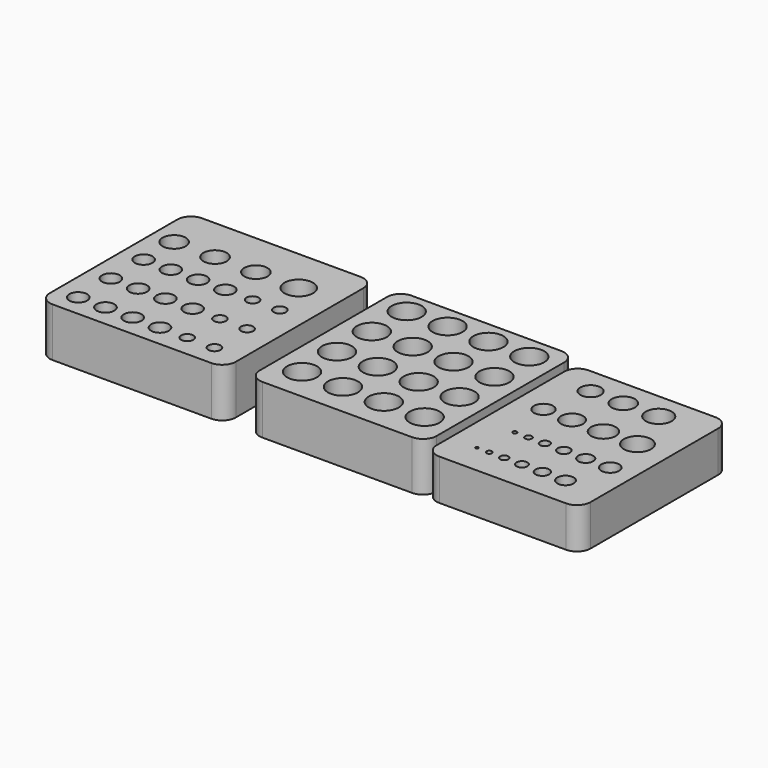
from build123d import *

# Parameters (mm, degrees)
F0_R     = 0.5
F0_R_2   = 1
F0_R_3   = 1.5
F0_R_4   = 2
F0_R_5   = 0.75
F0_R_6   = 1.25
F0_R_7   = 1.75
F0_R_8   = 2.5
F0_R_9   = 3
F0_R_10  = 2.25
F0_R_11  = 2.75
F0_R_12  = 3.25
F0_R_13  = 3.5
F0_R_14  = 4
F0_R_15  = 3.75
F0_R_16  = 4.25
F0_R_17  = 4.5
F0_R_18  = 5
F0_R_19  = 4.75
F1_DEPTH = 12
F2_DEPTH = 3
F3_R     = 5.5
F4_DEPTH = 15
F5_DEPTH = 3
F6_R     = 3.25
F6_R_2   = 2.25
F6_R_3   = 4.25
F6_R_4   = 5.25
F7_DEPTH = 15
F8_DEPTH = 3


with BuildPart() as f1:
    # F0 (on Top) → F1 (new body)
    with BuildSketch(Plane.XY):
        with BuildLine():
            Line((51.5, 68.5), (5, 68.5))
            ThreePointArc((5, 68.5), (1.4644660941, 67.0355339059), (0, 63.5))
            Line((0, 63.5), (0, 5))
            ThreePointArc((0, 5), (1.4644660941, 1.4644660941), (5, 0))
            Line((5, 0), (51.5, 0))
            ThreePointArc((51.5, 0), (55.0355339059, 1.4644660941), (56.5, 5))
            Line((56.5, 5), (56.5, 63.5))
            ThreePointArc((56.5, 63.5), (55.0355339059, 67.0355339059), (51.5, 68.5))
        make_face()
        with Locations((10, 11)):
            Circle(F0_R, mode=Mode.SUBTRACT)
        with Locations((14.5, 11)):
            Circle(F0_R_2, mode=Mode.SUBTRACT)
        with Locations((20, 11)):
            Circle(F0_R_3, mode=Mode.SUBTRACT)
        with Locations((26.5, 11)):
            Circle(F0_R_4, mode=Mode.SUBTRACT)
        with Locations((12.5, 25.25)):
            Circle(F0_R_5, mode=Mode.SUBTRACT)
        with Locations((17.5, 25.25)):
            Circle(F0_R_6, mode=Mode.SUBTRACT)
        with Locations((23.5, 25.25)):
            Circle(F0_R_7, mode=Mode.SUBTRACT)
        with Locations((34, 11)):
            Circle(F0_R_8, mode=Mode.SUBTRACT)
        with Locations((42.5, 11)):
            Circle(F0_R_9, mode=Mode.SUBTRACT)
        with Locations((30.5, 25.25)):
            Circle(F0_R_10, mode=Mode.SUBTRACT)
        with Locations((38.5, 25.25)):
            Circle(F0_R_11, mode=Mode.SUBTRACT)
        with Locations((47.5, 25.25)):
            Circle(F0_R_12, mode=Mode.SUBTRACT)
        with Locations((10, 41.5)):
            Circle(F0_R_13, mode=Mode.SUBTRACT)
        with Locations((20.5, 41.5)):
            Circle(F0_R_14, mode=Mode.SUBTRACT)
        with Locations((13.5, 58.75)):
            Circle(F0_R_15, mode=Mode.SUBTRACT)
        with Locations((25.5, 58.75)):
            Circle(F0_R_16, mode=Mode.SUBTRACT)
        with Locations((32, 41.5)):
            Circle(F0_R_17, mode=Mode.SUBTRACT)
        with Locations((44.5, 41.5)):
            Circle(F0_R_18, mode=Mode.SUBTRACT)
        with Locations((38.5, 58.75)):
            Circle(F0_R_19, mode=Mode.SUBTRACT)
    extrude(amount=F1_DEPTH)

    # F0 (on Top) → F2 (join)
    with BuildSketch(Plane.XY):
        with BuildLine():
            Line((51.5, 68.5), (5, 68.5))
            ThreePointArc((5, 68.5), (1.4644660941, 67.0355339059), (0, 63.5))
            Line((0, 63.5), (0, 5))
            ThreePointArc((0, 5), (1.4644660941, 1.4644660941), (5, 0))
            Line((5, 0), (51.5, 0))
            ThreePointArc((51.5, 0), (55.0355339059, 1.4644660941), (56.5, 5))
            Line((56.5, 5), (56.5, 63.5))
            ThreePointArc((56.5, 63.5), (55.0355339059, 67.0355339059), (51.5, 68.5))
        make_face()
        with Locations((10, 11)):
            Circle(F0_R, mode=Mode.SUBTRACT)
        with Locations((14.5, 11)):
            Circle(F0_R_2, mode=Mode.SUBTRACT)
        with Locations((20, 11)):
            Circle(F0_R_3, mode=Mode.SUBTRACT)
        with Locations((26.5, 11)):
            Circle(F0_R_4, mode=Mode.SUBTRACT)
        with Locations((12.5, 25.25)):
            Circle(F0_R_5, mode=Mode.SUBTRACT)
        with Locations((17.5, 25.25)):
            Circle(F0_R_6, mode=Mode.SUBTRACT)
        with Locations((23.5, 25.25)):
            Circle(F0_R_7, mode=Mode.SUBTRACT)
        with Locations((34, 11)):
            Circle(F0_R_8, mode=Mode.SUBTRACT)
        with Locations((42.5, 11)):
            Circle(F0_R_9, mode=Mode.SUBTRACT)
        with Locations((30.5, 25.25)):
            Circle(F0_R_10, mode=Mode.SUBTRACT)
        with Locations((38.5, 25.25)):
            Circle(F0_R_11, mode=Mode.SUBTRACT)
        with Locations((47.5, 25.25)):
            Circle(F0_R_12, mode=Mode.SUBTRACT)
        with Locations((10, 41.5)):
            Circle(F0_R_13, mode=Mode.SUBTRACT)
        with Locations((20.5, 41.5)):
            Circle(F0_R_14, mode=Mode.SUBTRACT)
        with Locations((13.5, 58.75)):
            Circle(F0_R_15, mode=Mode.SUBTRACT)
        with Locations((25.5, 58.75)):
            Circle(F0_R_16, mode=Mode.SUBTRACT)
        with Locations((32, 41.5)):
            Circle(F0_R_17, mode=Mode.SUBTRACT)
        with Locations((44.5, 41.5)):
            Circle(F0_R_18, mode=Mode.SUBTRACT)
        with Locations((38.5, 58.75)):
            Circle(F0_R_19, mode=Mode.SUBTRACT)
        with Locations((44.5, 41.5)):
            Circle(F0_R_18)
        with Locations((38.5, 58.75)):
            Circle(F0_R_19)
        with Locations((32, 41.5)):
            Circle(F0_R_17)
        with Locations((25.5, 58.75)):
            Circle(F0_R_16)
        with Locations((20.5, 41.5)):
            Circle(F0_R_14)
        with Locations((13.5, 58.75)):
            Circle(F0_R_15)
        with Locations((10, 41.5)):
            Circle(F0_R_13)
        with Locations((47.5, 25.25)):
            Circle(F0_R_12)
        with Locations((42.5, 11)):
            Circle(F0_R_9)
        with Locations((38.5, 25.25)):
            Circle(F0_R_11)
        with Locations((34, 11)):
            Circle(F0_R_8)
        with Locations((30.5, 25.25)):
            Circle(F0_R_10)
        with Locations((26.5, 11)):
            Circle(F0_R_4)
        with Locations((23.5, 25.25)):
            Circle(F0_R_7)
        with Locations((20, 11)):
            Circle(F0_R_3)
        with Locations((17.5, 25.25)):
            Circle(F0_R_6)
        with Locations((14.5, 11)):
            Circle(F0_R_2)
        with Locations((12.5, 25.25)):
            Circle(F0_R_5)
        with Locations((10, 11)):
            Circle(F0_R)
    extrude(amount=-F2_DEPTH)


with BuildPart() as f4:
    # F3 (on Top) → F4 (new body)
    with BuildSketch(Plane.XY):
        with BuildLine():
            Line((-60, 0), (-5, 0))
            ThreePointArc((-5, 0), (-1.4644660941, 1.4644660941), (0, 5))
            Line((0, 5), (0, 63.5))
            ThreePointArc((0, 63.5), (-1.4644660941, 67.0355339059), (-5, 68.5))
            Line((-5, 68.5), (-60, 68.5))
            ThreePointArc((-60, 68.5), (-63.5355339059, 67.0355339059), (-65, 63.5))
            Line((-65, 63.5), (-65, 5))
            ThreePointArc((-65, 5), (-63.5355339059, 1.4644660941), (-60, 0))
        make_face()
        with Locations((-55, 12)):
            Circle(F3_R, mode=Mode.SUBTRACT)
        with Locations((-40, 12)):
            Circle(F3_R, mode=Mode.SUBTRACT)
        with Locations((-55, 28)):
            Circle(F3_R, mode=Mode.SUBTRACT)
        with Locations((-40, 28)):
            Circle(F3_R, mode=Mode.SUBTRACT)
        with Locations((-25, 12)):
            Circle(F3_R, mode=Mode.SUBTRACT)
        with Locations((-10, 12)):
            Circle(F3_R, mode=Mode.SUBTRACT)
        with Locations((-25, 28)):
            Circle(F3_R, mode=Mode.SUBTRACT)
        with Locations((-10, 28)):
            Circle(F3_R, mode=Mode.SUBTRACT)
        with Locations((-55, 44)):
            Circle(F3_R, mode=Mode.SUBTRACT)
        with Locations((-40, 44)):
            Circle(F3_R, mode=Mode.SUBTRACT)
        with Locations((-55, 60)):
            Circle(F3_R, mode=Mode.SUBTRACT)
        with Locations((-40, 60)):
            Circle(F3_R, mode=Mode.SUBTRACT)
        with Locations((-25, 44)):
            Circle(F3_R, mode=Mode.SUBTRACT)
        with Locations((-10, 44)):
            Circle(F3_R, mode=Mode.SUBTRACT)
        with Locations((-25, 60)):
            Circle(F3_R, mode=Mode.SUBTRACT)
        with Locations((-10, 60)):
            Circle(F3_R, mode=Mode.SUBTRACT)
    extrude(amount=F4_DEPTH)

    # F3 (on Top) → F5 (join)
    with BuildSketch(Plane.XY):
        with BuildLine():
            Line((-60, 0), (-5, 0))
            ThreePointArc((-5, 0), (-1.4644660941, 1.4644660941), (0, 5))
            Line((0, 5), (0, 63.5))
            ThreePointArc((0, 63.5), (-1.4644660941, 67.0355339059), (-5, 68.5))
            Line((-5, 68.5), (-60, 68.5))
            ThreePointArc((-60, 68.5), (-63.5355339059, 67.0355339059), (-65, 63.5))
            Line((-65, 63.5), (-65, 5))
            ThreePointArc((-65, 5), (-63.5355339059, 1.4644660941), (-60, 0))
        make_face()
        with Locations((-55, 12)):
            Circle(F3_R, mode=Mode.SUBTRACT)
        with Locations((-40, 12)):
            Circle(F3_R, mode=Mode.SUBTRACT)
        with Locations((-55, 28)):
            Circle(F3_R, mode=Mode.SUBTRACT)
        with Locations((-40, 28)):
            Circle(F3_R, mode=Mode.SUBTRACT)
        with Locations((-25, 12)):
            Circle(F3_R, mode=Mode.SUBTRACT)
        with Locations((-10, 12)):
            Circle(F3_R, mode=Mode.SUBTRACT)
        with Locations((-25, 28)):
            Circle(F3_R, mode=Mode.SUBTRACT)
        with Locations((-10, 28)):
            Circle(F3_R, mode=Mode.SUBTRACT)
        with Locations((-55, 44)):
            Circle(F3_R, mode=Mode.SUBTRACT)
        with Locations((-40, 44)):
            Circle(F3_R, mode=Mode.SUBTRACT)
        with Locations((-55, 60)):
            Circle(F3_R, mode=Mode.SUBTRACT)
        with Locations((-40, 60)):
            Circle(F3_R, mode=Mode.SUBTRACT)
        with Locations((-25, 44)):
            Circle(F3_R, mode=Mode.SUBTRACT)
        with Locations((-10, 44)):
            Circle(F3_R, mode=Mode.SUBTRACT)
        with Locations((-25, 60)):
            Circle(F3_R, mode=Mode.SUBTRACT)
        with Locations((-10, 60)):
            Circle(F3_R, mode=Mode.SUBTRACT)
        with Locations((-55, 12)):
            Circle(F3_R)
        with Locations((-55, 28)):
            Circle(F3_R)
        with Locations((-55, 44)):
            Circle(F3_R)
        with Locations((-55, 60)):
            Circle(F3_R)
        with Locations((-40, 60)):
            Circle(F3_R)
        with Locations((-40, 44)):
            Circle(F3_R)
        with Locations((-40, 28)):
            Circle(F3_R)
        with Locations((-40, 12)):
            Circle(F3_R)
        with Locations((-25, 12)):
            Circle(F3_R)
        with Locations((-25, 28)):
            Circle(F3_R)
        with Locations((-25, 44)):
            Circle(F3_R)
        with Locations((-25, 60)):
            Circle(F3_R)
        with Locations((-10, 60)):
            Circle(F3_R)
        with Locations((-10, 44)):
            Circle(F3_R)
        with Locations((-10, 28)):
            Circle(F3_R)
        with Locations((-10, 12)):
            Circle(F3_R)
    extrude(amount=-F5_DEPTH)


with BuildPart() as f7:
    # F6 (on Top) → F7 (new body)
    with BuildSketch(Plane.XY):
        with BuildLine():
            Line((-136.9599341154, 0), (-78.7099341154, 0))
            ThreePointArc((-78.7099341154, 0), (-75.1744002095, 1.4644660941), (-73.7099341154, 5))
            Line((-73.7099341154, 5), (-73.7099341154, 63.5))
            ThreePointArc((-73.7099341154, 63.5), (-75.1744002095, 67.0355339059), (-78.7099341154, 68.5))
            Line((-78.7099341154, 68.5), (-136.9599341154, 68.5))
            ThreePointArc((-136.9599341154, 68.5), (-140.4954680213, 67.0355339059), (-141.9599341154, 63.5))
            Line((-141.9599341154, 63.5), (-141.9599341154, 5))
            ThreePointArc((-141.9599341154, 5), (-140.4954680213, 1.4644660941), (-136.9599341154, 0))
        make_face()
        with Locations((-133.9599341154, 8)):
            Circle(F6_R, mode=Mode.SUBTRACT)
        with Locations((-123.9599341154, 8)):
            Circle(F6_R, mode=Mode.SUBTRACT)
        with Locations((-113.9599341154, 8)):
            Circle(F6_R, mode=Mode.SUBTRACT)
        with Locations((-133.9599341154, 23)):
            Circle(F6_R, mode=Mode.SUBTRACT)
        with Locations((-123.9599341154, 23)):
            Circle(F6_R, mode=Mode.SUBTRACT)
        with Locations((-113.9599341154, 23)):
            Circle(F6_R, mode=Mode.SUBTRACT)
        with Locations((-103.9599341154, 8)):
            Circle(F6_R, mode=Mode.SUBTRACT)
        with Locations((-93.9599341154, 8)):
            Circle(F6_R_2, mode=Mode.SUBTRACT)
        with Locations((-83.9599341154, 8)):
            Circle(F6_R_2, mode=Mode.SUBTRACT)
        with Locations((-103.9599341154, 23)):
            Circle(F6_R, mode=Mode.SUBTRACT)
        with Locations((-93.9599341154, 23)):
            Circle(F6_R_2, mode=Mode.SUBTRACT)
        with Locations((-83.9599341154, 23)):
            Circle(F6_R_2, mode=Mode.SUBTRACT)
        with Locations((-133.9599341154, 38)):
            Circle(F6_R, mode=Mode.SUBTRACT)
        with Locations((-123.9599341154, 38)):
            Circle(F6_R, mode=Mode.SUBTRACT)
        with Locations((-113.9599341154, 38)):
            Circle(F6_R, mode=Mode.SUBTRACT)
        with Locations((-133.9599341154, 52.017354504)):
            Circle(F6_R_3, mode=Mode.SUBTRACT)
        with Locations((-118.9599341154, 52.017354504)):
            Circle(F6_R_3, mode=Mode.SUBTRACT)
        with Locations((-103.9599341154, 38)):
            Circle(F6_R, mode=Mode.SUBTRACT)
        with Locations((-93.9599341154, 38)):
            Circle(F6_R_2, mode=Mode.SUBTRACT)
        with Locations((-83.9599341154, 38)):
            Circle(F6_R_2, mode=Mode.SUBTRACT)
        with Locations((-103.9599341154, 52.017354504)):
            Circle(F6_R_3, mode=Mode.SUBTRACT)
        with Locations((-88.2544073784, 52.017354504)):
            Circle(F6_R_4, mode=Mode.SUBTRACT)
    extrude(amount=F7_DEPTH)

    # F6 (on Top) → F8 (join)
    with BuildSketch(Plane.XY):
        with BuildLine():
            Line((-136.9599341154, 0), (-78.7099341154, 0))
            ThreePointArc((-78.7099341154, 0), (-75.1744002095, 1.4644660941), (-73.7099341154, 5))
            Line((-73.7099341154, 5), (-73.7099341154, 63.5))
            ThreePointArc((-73.7099341154, 63.5), (-75.1744002095, 67.0355339059), (-78.7099341154, 68.5))
            Line((-78.7099341154, 68.5), (-136.9599341154, 68.5))
            ThreePointArc((-136.9599341154, 68.5), (-140.4954680213, 67.0355339059), (-141.9599341154, 63.5))
            Line((-141.9599341154, 63.5), (-141.9599341154, 5))
            ThreePointArc((-141.9599341154, 5), (-140.4954680213, 1.4644660941), (-136.9599341154, 0))
        make_face()
        with Locations((-133.9599341154, 8)):
            Circle(F6_R, mode=Mode.SUBTRACT)
        with Locations((-123.9599341154, 8)):
            Circle(F6_R, mode=Mode.SUBTRACT)
        with Locations((-113.9599341154, 8)):
            Circle(F6_R, mode=Mode.SUBTRACT)
        with Locations((-133.9599341154, 23)):
            Circle(F6_R, mode=Mode.SUBTRACT)
        with Locations((-123.9599341154, 23)):
            Circle(F6_R, mode=Mode.SUBTRACT)
        with Locations((-113.9599341154, 23)):
            Circle(F6_R, mode=Mode.SUBTRACT)
        with Locations((-103.9599341154, 8)):
            Circle(F6_R, mode=Mode.SUBTRACT)
        with Locations((-93.9599341154, 8)):
            Circle(F6_R_2, mode=Mode.SUBTRACT)
        with Locations((-83.9599341154, 8)):
            Circle(F6_R_2, mode=Mode.SUBTRACT)
        with Locations((-103.9599341154, 23)):
            Circle(F6_R, mode=Mode.SUBTRACT)
        with Locations((-93.9599341154, 23)):
            Circle(F6_R_2, mode=Mode.SUBTRACT)
        with Locations((-83.9599341154, 23)):
            Circle(F6_R_2, mode=Mode.SUBTRACT)
        with Locations((-133.9599341154, 38)):
            Circle(F6_R, mode=Mode.SUBTRACT)
        with Locations((-123.9599341154, 38)):
            Circle(F6_R, mode=Mode.SUBTRACT)
        with Locations((-113.9599341154, 38)):
            Circle(F6_R, mode=Mode.SUBTRACT)
        with Locations((-133.9599341154, 52.017354504)):
            Circle(F6_R_3, mode=Mode.SUBTRACT)
        with Locations((-118.9599341154, 52.017354504)):
            Circle(F6_R_3, mode=Mode.SUBTRACT)
        with Locations((-103.9599341154, 38)):
            Circle(F6_R, mode=Mode.SUBTRACT)
        with Locations((-93.9599341154, 38)):
            Circle(F6_R_2, mode=Mode.SUBTRACT)
        with Locations((-83.9599341154, 38)):
            Circle(F6_R_2, mode=Mode.SUBTRACT)
        with Locations((-103.9599341154, 52.017354504)):
            Circle(F6_R_3, mode=Mode.SUBTRACT)
        with Locations((-88.2544073784, 52.017354504)):
            Circle(F6_R_4, mode=Mode.SUBTRACT)
        with Locations((-88.2544073784, 52.017354504)):
            Circle(F6_R_4)
        with Locations((-133.9599341154, 52.017354504)):
            Circle(F6_R_3)
        with Locations((-118.9599341154, 52.017354504)):
            Circle(F6_R_3)
        with Locations((-103.9599341154, 52.017354504)):
            Circle(F6_R_3)
        with Locations((-103.9599341154, 38)):
            Circle(F6_R)
        with Locations((-123.9599341154, 38)):
            Circle(F6_R)
        with Locations((-133.9599341154, 38)):
            Circle(F6_R)
        with Locations((-133.9599341154, 23)):
            Circle(F6_R)
        with Locations((-123.9599341154, 23)):
            Circle(F6_R)
        with Locations((-113.9599341154, 23)):
            Circle(F6_R)
        with Locations((-103.9599341154, 23)):
            Circle(F6_R)
        with Locations((-103.9599341154, 8)):
            Circle(F6_R)
        with Locations((-113.9599341154, 8)):
            Circle(F6_R)
        with Locations((-123.9599341154, 8)):
            Circle(F6_R)
        with Locations((-133.9599341154, 8)):
            Circle(F6_R)
        with Locations((-113.9599341154, 38)):
            Circle(F6_R)
        with Locations((-83.9599341154, 38)):
            Circle(F6_R_2)
        with Locations((-93.9599341154, 38)):
            Circle(F6_R_2)
        with Locations((-93.9599341154, 23)):
            Circle(F6_R_2)
        with Locations((-83.9599341154, 23)):
            Circle(F6_R_2)
        with Locations((-83.9599341154, 8)):
            Circle(F6_R_2)
        with Locations((-93.9599341154, 8)):
            Circle(F6_R_2)
    extrude(amount=-F8_DEPTH)


solid = Compound([f1.part, f4.part, f7.part])
